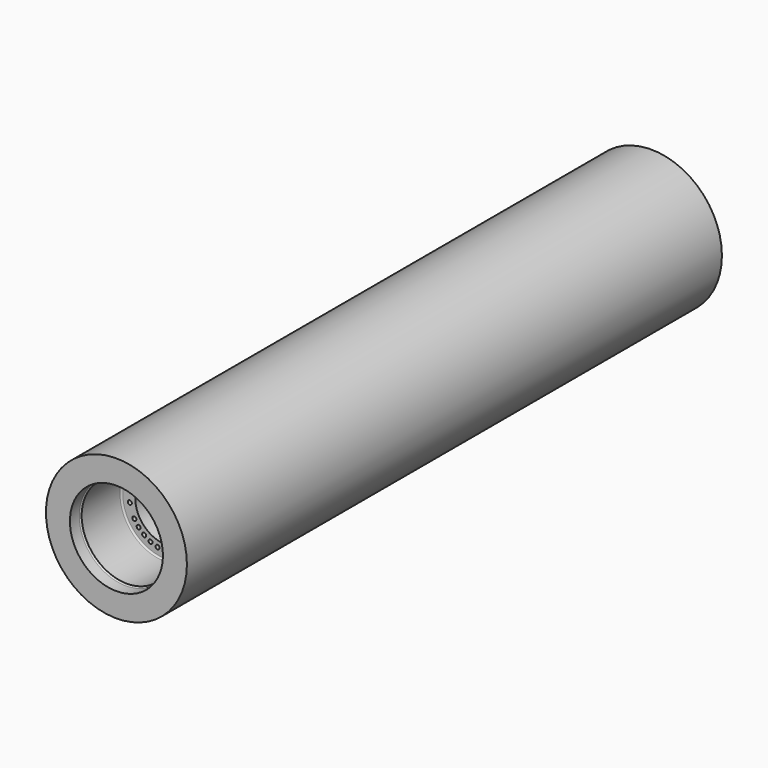
from build123d import *

# Parameters (mm, degrees)
F0_R      = 135.89
F1_DEPTH  = 1289.304
F2_R      = 87.376
F3_DEPTH  = 120.65
F4_R      = 89.662
F5_DEPTH  = 25.4
F6_R      = 60.325
F7_DEPTH  = 1397
F9_R      = 3.937
F10_DEPTH = 762
F11_DEPTH = 762


# Not quite as in the source:
# - a fillet or chamfer that OpenCascade refuses, or shapes differently, is made with other operations: its cross-section is extruded or revolved along the edge and cut away or added


with BuildPart() as f1:
    # F0 (on Front) → F1 (new body)
    with BuildSketch(Plane.XZ):
        Circle(F0_R)
    extrude(amount=F1_DEPTH)

    # F2 (on face) → F3 (cut)
    with BuildSketch(Plane.XZ.offset(1289.304)):
        Circle(F2_R)
    extrude(amount=-F3_DEPTH, mode=Mode.SUBTRACT)

    # F4 (on face) → F5 (cut)
    with BuildSketch(Plane.XZ.offset(1289.304)):
        Circle(F4_R)
    extrude(amount=-F5_DEPTH, mode=Mode.SUBTRACT)

    # F6 (on face) → F7 (cut)
    with BuildSketch(Plane.XZ.offset(1168.654)):
        Circle(F6_R)
    extrude(amount=-F7_DEPTH, mode=Mode.SUBTRACT)

    # F8: fillet of radius 3.048 on 2 edges, made by hand

    # F8_s1 → F8_t2 (revolve)
    with BuildSketch(Plane.XY):
        with BuildLine():
            ThreePointArc((84.328, -1168.654), (86.4832614691, -1169.5467385309), (87.376, -1171.702))
            Line((87.376, -1171.702), (87.376, -1168.654))
            Line((87.376, -1168.654), (84.328, -1168.654))
        make_face()
    revolve(axis=Axis((0, -1168.654, 0), (0, -1, 0)))

    # F8_s3 → F8_t4 (revolve)
    with BuildSketch(Plane.XY):
        with BuildLine():
            ThreePointArc((89.662, -1266.8552133098), (89.023655577, -1264.9887021258), (87.376, -1263.904))
            Line((87.376, -1263.904), (89.662, -1263.904))
            Line((89.662, -1263.904), (89.662, -1266.8552133098))
        make_face()
    revolve(axis=Axis((0, -1263.904, 0), (0, -1, 0)))

    # F9 (on face) → F10 (cut)
    with BuildSketch(Plane.XZ.offset(1168.654)):
        with Locations((-60.0598781159, 39.003340895)):
            Circle(F9_R)
        with Locations((-43.0978960277, 58.6797422495)):
            Circle(F9_R)
        with Locations((-18.5348584976, 69.173033624)):
            Circle(F9_R)
        with Locations((-70.0482739288, 14.8892202572)):
            Circle(F9_R)
        with Locations((-70.7315167837, -11.2027716991)):
            Circle(F9_R)
        with Locations((-62.0188452827, -35.8065970188)):
            Circle(F9_R)
        with Locations((-53.6351113584, -47.4523380861)):
            Circle(F9_R)
        with Locations((-43.0978960277, -57.1928397463)):
            Circle(F9_R)
        with Locations((-30.8302747111, -64.6370151036)):
            Circle(F9_R)
        with Locations((-17.3247996515, -69.4859761197)):
            Circle(F9_R)
        with Locations((-3.1237236512, -71.5450341451)):
            Circle(F9_R)
        with Locations((11.2027716991, -70.7315167837)):
            Circle(F9_R)
        with Locations((37.9492110938, -60.7314328633)):
            Circle(F9_R)
        with Locations((53.218974585, -47.9185799497)):
            Circle(F9_R)
        with Locations((66.8566762325, -25.6638735077)):
            Circle(F9_R)
        with Locations((71.6131940376, 0)):
            Circle(F9_R)
        with Locations((66.8566762325, 25.6638735077)):
            Circle(F9_R)
        with Locations((32.5117097491, 63.8078231055)):
            Circle(F9_R)
    extrude(amount=-F10_DEPTH, mode=Mode.SUBTRACT)

    # F9 (on face) → F11 (cut)
    with BuildSketch(Plane.XZ.offset(1168.654)):
        with Locations((-60.0598781159, 39.003340895)):
            Circle(F9_R)
        with Locations((-43.0978960277, 58.6797422495)):
            Circle(F9_R)
        with Locations((-18.5348584976, 69.173033624)):
            Circle(F9_R)
        with Locations((-70.0482739288, 14.8892202572)):
            Circle(F9_R)
        with Locations((-70.7315167837, -11.2027716991)):
            Circle(F9_R)
        with Locations((-62.0188452827, -35.8065970188)):
            Circle(F9_R)
        with Locations((-53.6351113584, -47.4523380861)):
            Circle(F9_R)
        with Locations((-43.0978960277, -57.1928397463)):
            Circle(F9_R)
        with Locations((-30.8302747111, -64.6370151036)):
            Circle(F9_R)
        with Locations((-17.3247996515, -69.4859761197)):
            Circle(F9_R)
        with Locations((-3.1237236512, -71.5450341451)):
            Circle(F9_R)
        with Locations((11.2027716991, -70.7315167837)):
            Circle(F9_R)
        with Locations((37.9492110938, -60.7314328633)):
            Circle(F9_R)
        with Locations((53.218974585, -47.9185799497)):
            Circle(F9_R)
        with Locations((66.8566762325, -25.6638735077)):
            Circle(F9_R)
        with Locations((71.6131940376, 0)):
            Circle(F9_R)
        with Locations((66.8566762325, 25.6638735077)):
            Circle(F9_R)
        with Locations((32.5117097491, 63.8078231055)):
            Circle(F9_R)
    extrude(amount=-F11_DEPTH, mode=Mode.SUBTRACT)


solid = f1.part
